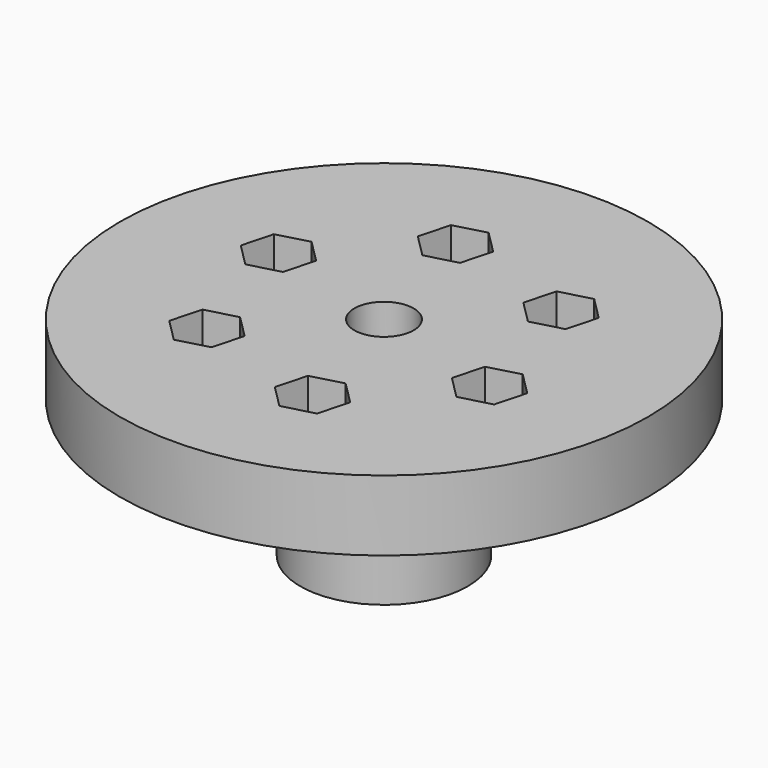
from build123d import *

# Parameters (mm, degrees)
F0_R      = 45.212
F1_DEPTH  = 12.065
F2_R      = 2.5908
F3_DEPTH  = 25.4
F4_R      = 14.5415
F5_DEPTH  = 25.4
F7_DEPTH  = 9.525
F8_R      = 15.24
F9_DEPTH  = 12.065
F10_R     = 14.351
F11_DEPTH = 35.56
F12_R     = 5.08
F13_DEPTH = 38.1


# Not quite as in the source:
# - a feature names something its author has since deleted; it is built from what else it names


with BuildPart() as f1:
    # F0 (on Top) → F1 (new body)
    with BuildSketch(Plane.XY):
        Circle(F0_R)
    extrude(amount=F1_DEPTH)

    # F2 (on face) → F3 (cut)
    with BuildSketch(Plane.XY.offset(12.065)):
        with Locations((-6.1631285115, 23.0011087385)):
            Circle(F2_R)
        with Locations((-23.0011087385, 6.1631285115)):
            Circle(F2_R)
        with Locations((-16.837980227, -16.837980227)):
            Circle(F2_R)
        with Locations((6.1631285115, -23.0011087385)):
            Circle(F2_R)
        with Locations((23.0011087385, -6.1631285115)):
            Circle(F2_R)
        with Locations((16.837980227, 16.837980227)):
            Circle(F2_R)
    extrude(amount=-F3_DEPTH, mode=Mode.SUBTRACT)

    # F4 (on face) → F5 (cut)
    with BuildSketch(Plane.XY.offset(12.065)):
        Circle(F4_R)
    extrude(amount=-F5_DEPTH, mode=Mode.SUBTRACT)

    # F6 (on face) → F7 (cut)
    with BuildSketch(Plane.XY.offset(12.065)):
        Polygon((-4.7398149494, 28.3129872672), (-10.0516934782, 26.8896737052), (-11.4750070402, 21.5777951764), (-7.5864420736, 17.6892302098), (-2.2745635448, 19.1125437718), (-0.8512499828, 24.4244223006), align=None)
        Polygon((22.1498587557, 18.2612937891), (18.2612937891, 22.1498587557), (12.9494152603, 20.7265451937), (11.5261016983, 15.4146666649), (15.4146666649, 11.5261016983), (20.7265451937, 12.9494152603), align=None)
        Polygon((26.8896737052, -10.0516934782), (28.3129872672, -4.7398149494), (24.4244223006, -0.8512499828), (19.1125437718, -2.2745635448), (17.6892302098, -7.5864420736), (21.5777951764, -11.4750070402), align=None)
        Polygon((4.7398149494, -28.3129872672), (10.0516934782, -26.8896737052), (11.4750070402, -21.5777951764), (7.5864420736, -17.6892302098), (2.2745635448, -19.1125437718), (0.8512499828, -24.4244223006), align=None)
        Polygon((-22.1498587557, -18.2612937891), (-18.2612937891, -22.1498587557), (-12.9494152603, -20.7265451937), (-11.5261016983, -15.4146666649), (-15.4146666649, -11.5261016983), (-20.7265451937, -12.9494152603), align=None)
        Polygon((-26.8896737052, 10.0516934782), (-28.3129872672, 4.7398149494), (-24.4244223006, 0.8512499828), (-19.1125437718, 2.2745635448), (-17.6892302098, 7.5864420736), (-21.5777951764, 11.4750070402), align=None)
    extrude(amount=-F7_DEPTH, mode=Mode.SUBTRACT)

    # F8 (on face) → F9 (join)
    with BuildSketch(Plane.XY.offset(12.065)):
        Circle(F8_R)
    extrude(amount=-F9_DEPTH)

    # F10 (on face) → F11 (join)
    with BuildSketch(Plane.XY.offset(12.065)):
        Circle(F10_R)
    extrude(amount=-F11_DEPTH)

    # F12 (on face) → F13 (cut)
    with BuildSketch(Plane.XY.offset(12.065)):
        Circle(F12_R)
    extrude(amount=-F13_DEPTH, mode=Mode.SUBTRACT)


solid = f1.part
